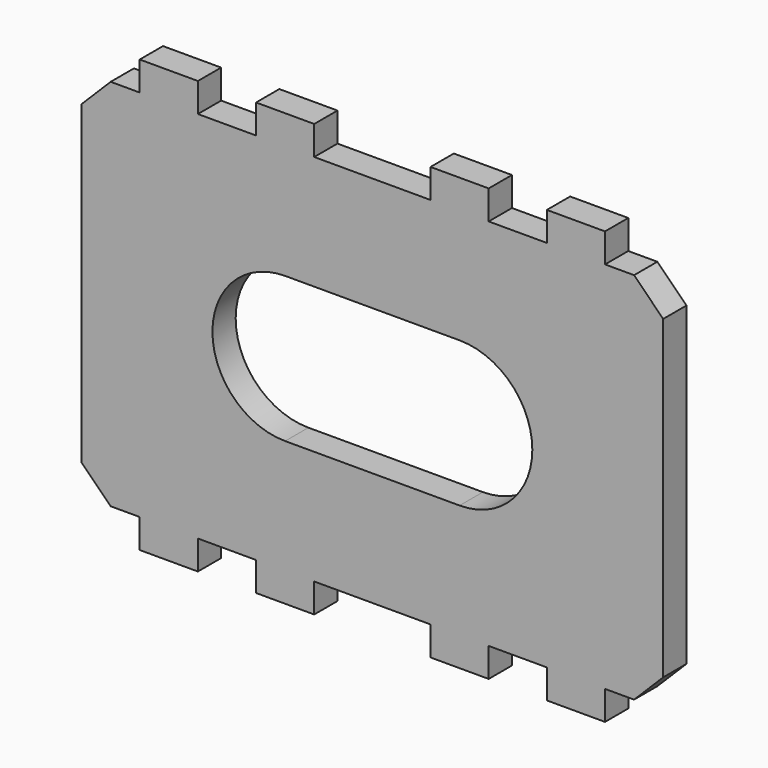
from build123d import *

# Parameters (mm, degrees)
F0_W     = 100
F0_H     = 64.25
F1_DEPTH = 5
F2_SIZE  = 5
F3_W     = 10
F3_H     = 5
F4_DEPTH = 5


# Not quite as in the source:
# - a pattern or mirror of a feature is missing from the dataset's text; its kind, count and spacing are read off the source's solid


with BuildPart() as f1:
    # F0 (on Front) → F1 (new body)
    with BuildSketch(Plane.XZ):
        Rectangle(F0_W, F0_H)
        with BuildLine():
            Line((15, -12.5), (-15, -12.5))
            ThreePointArc((-15, -12.5), (-27.5, 0), (-15, 12.5))
            Line((-15, 12.5), (15, 12.5))
            ThreePointArc((15, 12.5), (27.5, 0), (15, -12.5))
        make_face(mode=Mode.SUBTRACT)
    extrude(amount=F1_DEPTH)

    # F2
    f2_edges = [f1.edges().sort_by_distance(p)[0] for p in [
        (-50, -2.5, 32.125),
        (50, -2.5, 32.125),
        (-50, -2.5, -32.125),
        (50, -2.5, -32.125),
    ]]
    chamfer(f2_edges, length=F2_SIZE)

    # F3 (on face) → F4 (join)
    with BuildSketch(Plane(origin=(0, 0, -32.125), x_dir=(1, 0, 0), z_dir=(0, 0, -1))):
        with Locations((35, 2.5)):
            Rectangle(F3_W, F3_H)
        with Locations((15, 2.5)):
            Rectangle(F3_W, F3_H)
        with Locations((-15, 2.5)):
            Rectangle(F3_W, F3_H)
        with Locations((-35, 2.5)):
            Rectangle(F3_W, F3_H)
    f4 = extrude(amount=F4_DEPTH)

    # F4_copies: F4 across plane
    add(f4.mirror(Plane.XY))


solid = f1.part
